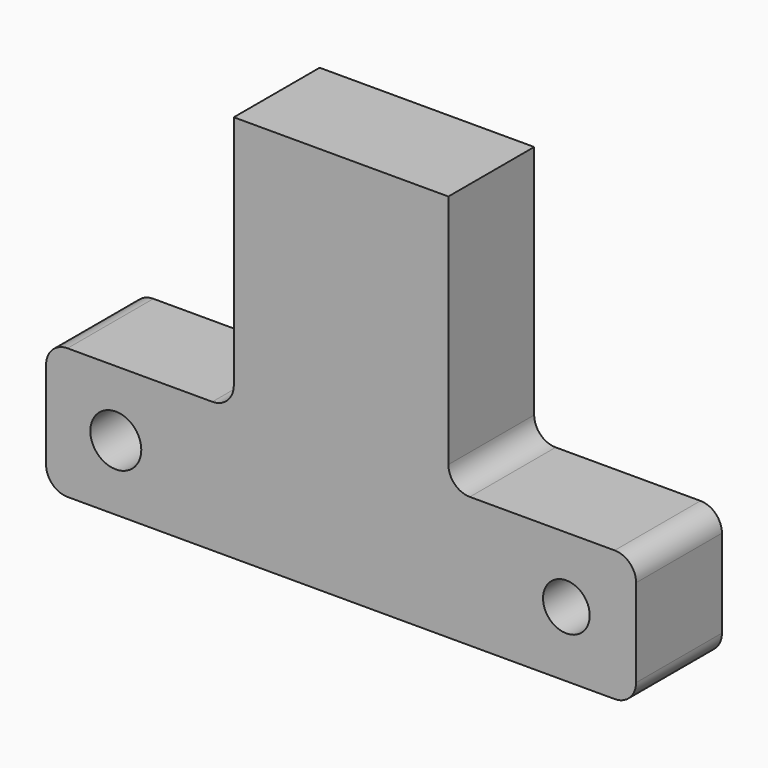
from build123d import *

# Parameters (mm, degrees)
F0_W     = 55
F0_H     = 12.2
F0_R     = 2.374951393
F0_R_2   = 2.1771962512
F1_DEPTH = 10
F2_W     = 20
F2_H     = 10
F3_DEPTH = 24
F4_R     = 2


with BuildPart() as f1:
    # F0 (on Front) → F1 (new body)
    with BuildSketch(Plane.XZ):
        Rectangle(F0_W, F0_H)
        with Locations((-21, 0)):
            Circle(F0_R, mode=Mode.SUBTRACT)
        with Locations((21, 0)):
            Circle(F0_R_2, mode=Mode.SUBTRACT)
    extrude(amount=F1_DEPTH)

    # F2 (on face) → F3 (join)
    with BuildSketch(Plane.XY.offset(6.1)):
        with Locations((0, -5)):
            Rectangle(F2_W, F2_H)
    extrude(amount=F3_DEPTH)

    # F4
    f4_edges = [f1.edges().sort_by_distance(p)[0] for p in [
        (10, -5, 6.1),
        (27.5, -5, 6.1),
        (27.5, -5, -6.1),
        (-10, -5, 6.1),
        (-27.5, -5, 6.1),
        (-27.5, -5, -6.1),
    ]]
    fillet(f4_edges, radius=F4_R)


solid = f1.part
